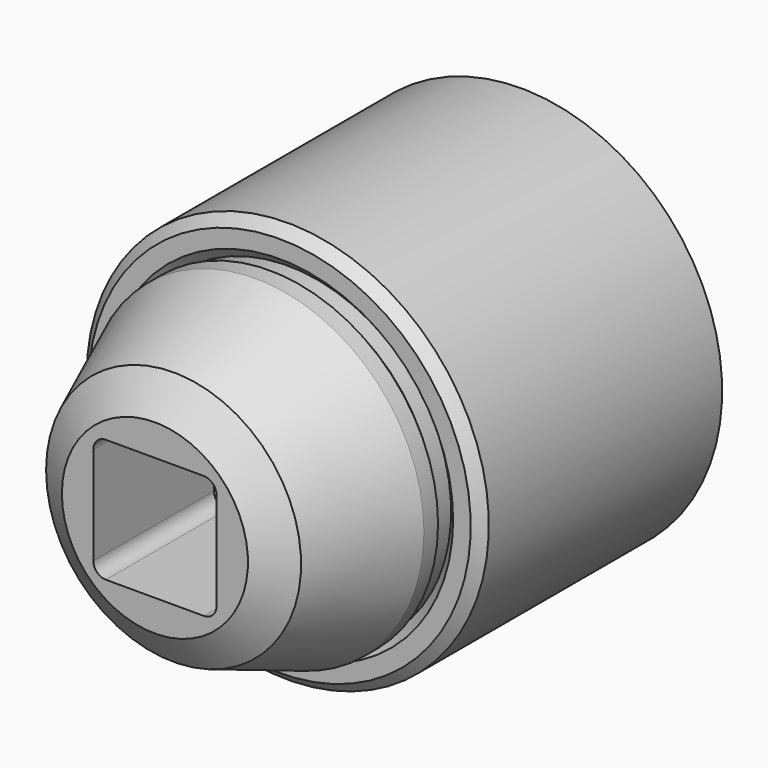
from build123d import *
from build123d import SkipClean  # not in build123d's __all__

# Parameters (mm, degrees)
F1_DEPTH   = 24.4
F2_DEPTH   = 12
F3_R       = 1
F4_DEPTH   = 24.4
F5_SIZE2   = 4
F5_SIZE    = 10
F7_R       = 13.4
F7_R_2     = 12.6
F8_DEPTH   = 22
F11_SIZE   = 2
F10_R      = 16
F10_R_2    = 14.2
F10_R_3    = 13
F12_DEPTH  = 20
F13_DEPTH  = 4
F14_SIZE   = 0.79999
F14_2_SIZE = 0.79999
F15_R      = 1


# Not quite as in the source:
# - two fillets or chamfers of one size are made in one step
# - a fillet or chamfer is up to 0.001 mm smaller than in the source, because OpenCascade refuses the exact size
# - after a boolean that leaves OpenCascade's solid faulty, fix() repairs it


with BuildPart() as f1:
    # F0 (on Front) → F1 (new body)
    with BuildSketch(Plane.XZ):
        with BuildLine():
            Line((12.1, -2.5), (10.0950482911, -2.5))
            ThreePointArc((10.0950482911, -2.5), (0, -10.4), (-10.0950482911, -2.5))
            Line((-10.0950482911, -2.5), (-12.1, -2.5))
            Line((-12.1, -2.5), (-12.1, 0))
            Line((-12.1, 0), (-13.4, 0))
            ThreePointArc((-13.4, 0), (0, -13.4), (13.4, 0))
            Line((13.4, 0), (12.1, 0))
            Line((12.1, 0), (12.1, -2.5))
        make_face()
        with BuildLine():
            ThreePointArc((-10.0950482911, 2.5), (0, 10.4), (10.0950482911, 2.5))
            Line((10.0950482911, 2.5), (12.1, 2.5))
            Line((12.1, 2.5), (12.1, 0))
            Line((12.1, 0), (13.4, 0))
            ThreePointArc((13.4, 0), (0, 13.4), (-13.4, 0))
            Line((-13.4, 0), (-12.1, 0))
            Line((-12.1, 0), (-12.1, 2.5))
            Line((-12.1, 2.5), (-10.0950482911, 2.5))
        make_face()
    extrude(amount=-F1_DEPTH)

    # F0 (on Front) → F2 (join)
    with BuildSketch(Plane.XZ):
        with BuildLine():
            Line((4.9, 0), (8.1, 0))
            ThreePointArc((8.1, 0), (0, 8.1), (-8.1, 0))
            Line((-8.1, 0), (-4.9, 0))
            Line((-4.9, 0), (-4.9, 4.9))
            Line((-4.9, 4.9), (4.9, 4.9))
            Line((4.9, 4.9), (4.9, 0))
        make_face()
        with BuildLine():
            Line((8.1, 0), (10.4, 0))
            ThreePointArc((10.4, 0), (10.3234805717, 1.2592652168), (10.0950482911, 2.5))
            ThreePointArc((10.0950482911, 2.5), (0, 10.4), (-10.0950482911, 2.5))
            ThreePointArc((-10.0950482911, 2.5), (-10.3234805717, 1.2592652168), (-10.4, 0))
            Line((-10.4, 0), (-8.1, 0))
            ThreePointArc((-8.1, 0), (0, 8.1), (8.1, 0))
        make_face()
        with BuildLine():
            ThreePointArc((-10.0950482911, 2.5), (0, 10.4), (10.0950482911, 2.5))
            Line((10.0950482911, 2.5), (12.1, 2.5))
            Line((12.1, 2.5), (12.1, 0))
            Line((12.1, 0), (13.4, 0))
            ThreePointArc((13.4, 0), (0, 13.4), (-13.4, 0))
            Line((-13.4, 0), (-12.1, 0))
            Line((-12.1, 0), (-12.1, 2.5))
            Line((-12.1, 2.5), (-10.0950482911, 2.5))
        make_face()
        with BuildLine():
            ThreePointArc((-8.1, 0), (0, -8.1), (8.1, 0))
            Line((8.1, 0), (4.9, 0))
            Line((4.9, 0), (4.9, -4.9))
            Line((4.9, -4.9), (-4.9, -4.9))
            Line((-4.9, -4.9), (-4.9, 0))
            Line((-4.9, 0), (-8.1, 0))
        make_face()
        with BuildLine():
            ThreePointArc((10.0950482911, -2.5), (10.3234805717, -1.2592652168), (10.4, 0))
            Line((10.4, 0), (8.1, 0))
            ThreePointArc((8.1, 0), (0, -8.1), (-8.1, 0))
            Line((-8.1, 0), (-10.4, 0))
            ThreePointArc((-10.4, 0), (-10.3234805717, -1.2592652168), (-10.0950482911, -2.5))
            ThreePointArc((-10.0950482911, -2.5), (0, -10.4), (10.0950482911, -2.5))
        make_face()
        with BuildLine():
            Line((12.1, -2.5), (10.0950482911, -2.5))
            ThreePointArc((10.0950482911, -2.5), (0, -10.4), (-10.0950482911, -2.5))
            Line((-10.0950482911, -2.5), (-12.1, -2.5))
            Line((-12.1, -2.5), (-12.1, 0))
            Line((-12.1, 0), (-13.4, 0))
            ThreePointArc((-13.4, 0), (0, -13.4), (13.4, 0))
            Line((13.4, 0), (12.1, 0))
            Line((12.1, 0), (12.1, -2.5))
        make_face()
        with BuildLine():
            Line((12.1, 0), (10.4, 0))
            ThreePointArc((10.4, 0), (10.3234805717, -1.2592652168), (10.0950482911, -2.5))
            Line((10.0950482911, -2.5), (12.1, -2.5))
            Line((12.1, -2.5), (12.1, 0))
        make_face()
        with BuildLine():
            ThreePointArc((10.0950482911, 2.5), (10.3234805717, 1.2592652168), (10.4, 0))
            Line((10.4, 0), (12.1, 0))
            Line((12.1, 0), (12.1, 2.5))
            Line((12.1, 2.5), (10.0950482911, 2.5))
        make_face()
        with BuildLine():
            Line((-12.1, -2.5), (-10.0950482911, -2.5))
            ThreePointArc((-10.0950482911, -2.5), (-10.3234805717, -1.2592652168), (-10.4, 0))
            Line((-10.4, 0), (-12.1, 0))
            Line((-12.1, 0), (-12.1, -2.5))
        make_face()
        with BuildLine():
            ThreePointArc((-10.4, 0), (-10.3234805717, 1.2592652168), (-10.0950482911, 2.5))
            Line((-10.0950482911, 2.5), (-12.1, 2.5))
            Line((-12.1, 2.5), (-12.1, 0))
            Line((-12.1, 0), (-10.4, 0))
        make_face()
    with SkipClean():  # cleaning this boolean's faces spoils the solid; the shape is the same uncleaned
        extrude(amount=F2_DEPTH)

    # F3
    f3_edges = [f1.edges().sort_by_distance(p)[0] for p in [
        (-4.9, -6, 4.9),
        (4.9, -6, 4.9),
        (4.9, -6, -4.9),
        (-4.9, -6, -4.9),
    ]]
    fillet(f3_edges, radius=F3_R)

    # F0 (on Front) → F4 (join, through all)
    with BuildSketch(Plane.XZ):
        with BuildLine():
            Line((12.1, 0), (10.4, 0))
            ThreePointArc((10.4, 0), (10.3234805717, -1.2592652168), (10.0950482911, -2.5))
            Line((10.0950482911, -2.5), (12.1, -2.5))
            Line((12.1, -2.5), (12.1, 0))
        make_face()
        with BuildLine():
            ThreePointArc((10.0950482911, -2.5), (10.3234805717, -1.2592652168), (10.4, 0))
            Line((10.4, 0), (8.1, 0))
            ThreePointArc((8.1, 0), (0, -8.1), (-8.1, 0))
            Line((-8.1, 0), (-10.4, 0))
            ThreePointArc((-10.4, 0), (-10.3234805717, -1.2592652168), (-10.0950482911, -2.5))
            ThreePointArc((-10.0950482911, -2.5), (0, -10.4), (10.0950482911, -2.5))
        make_face()
        with BuildLine():
            Line((-12.1, -2.5), (-10.0950482911, -2.5))
            ThreePointArc((-10.0950482911, -2.5), (-10.3234805717, -1.2592652168), (-10.4, 0))
            Line((-10.4, 0), (-12.1, 0))
            Line((-12.1, 0), (-12.1, -2.5))
        make_face()
    extrude(amount=-F4_DEPTH)

    add(f1.part.fix(), mode=Mode.REPLACE)

    # F5
    f5_edges = [f1.edges().sort_by_distance(p)[0] for p in [
        (13.4, -12, 0),
    ]]
    f5_side = f1.faces().sort_by_distance((13.4, -6, 0))[0]
    chamfer(f5_edges, length=F5_SIZE, length2=F5_SIZE2, reference=f5_side)

    # F7 (on offset) → F8 (cut)
    with BuildSketch(Plane(origin=(0, 21.4, 0), x_dir=(-1, 0, 0), z_dir=(0, 1, 0))):
        Circle(F7_R)
        Circle(F7_R_2, mode=Mode.SUBTRACT)
    extrude(amount=-F8_DEPTH, mode=Mode.SUBTRACT)

    # F11
    f11_edges = [f1.edges().sort_by_distance(p)[0] for p in [
        (9.4, -12, 0),
    ]]
    chamfer(f11_edges, length=F11_SIZE)

    # F14 (size 0.8 in the source; OpenCascade refuses exactly that, so slightly less here)
    f14_edges = [f1.edges().sort_by_distance(p)[0] for p in [
        (-13.4, 21.4, 0),
        (12.6, -0.6, 0),
    ]]
    chamfer(f14_edges, length=F14_SIZE)

    # F15
    f15_edges = [f1.edges().sort_by_distance(p)[0] for p in [
        (8.1, 12.2, 0),
        (-8.1, 12.2, 0),
        (10.1, 24.4, 0),
        (0, 24.4, -8.1),
        (-10.1, 24.4, 0),
        (-11.097524, 24.4, 2.5),
        (0, 24.4, 10.4),
        (11.097524, 24.4, 2.5),
        (-10.095048, 12.2, 2.5),
        (10.095048, 12.2, 2.5),
    ]]
    fillet(f15_edges, radius=F15_R)


with BuildPart() as f12:
    # F10 (on offset) → F12 (new body)
    with BuildSketch(Plane(origin=(0, 20.4, 0), x_dir=(-1, 0, 0), z_dir=(0, 1, 0))):
        Circle(F10_R)
        Circle(F10_R_2, mode=Mode.SUBTRACT)
        Circle(F10_R_2)
        Circle(F10_R_3, mode=Mode.SUBTRACT)
    extrude(amount=-F12_DEPTH)

    # F10 (on offset) → F13 (join, through all)
    with BuildSketch(Plane(origin=(0, 20.4, 0), x_dir=(-1, 0, 0), z_dir=(0, 1, 0))):
        Circle(F10_R)
        Circle(F10_R_2, mode=Mode.SUBTRACT)
    extrude(amount=F13_DEPTH)

    # F14#2 (size 0.8 in the source; OpenCascade refuses exactly that, so slightly less here)
    f14_2_edges = [f12.edges().sort_by_distance(p)[0] for p in [
        (16, 0.4, 0),
        (14.2, 20.4, 0),
        (13, 0.4, 0),
    ]]
    chamfer(f14_2_edges, length=F14_2_SIZE)


solid = Compound([f1.part, f12.part])
